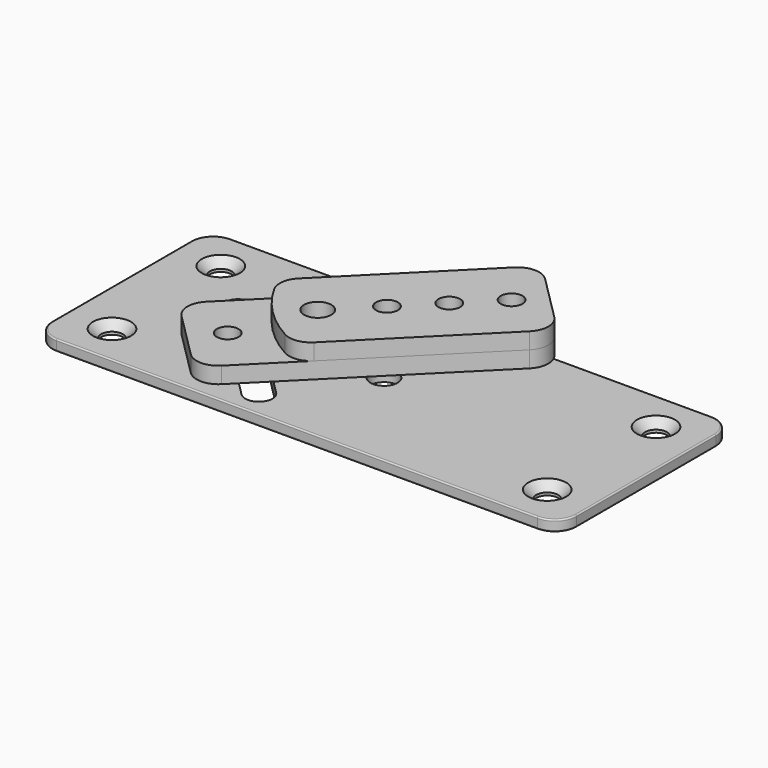
from build123d import *

# Parameters (mm, degrees)
F0_W      = 96.4
F0_H      = 2
F1_DEPTH  = 20
F2_R      = 4
F3_R      = 0.25
F4_R      = 2
F4_R_2    = 2.5
F5_DEPTH  = 2.0010001
F6_SIZE   = 1.5
F8_DEPTH  = 2.0010001
F9_R      = 2
F10_DEPTH = 3
F11_R     = 2.5
F11_R_2   = 2
F12_DEPTH = 3


# Not quite as in the source:
# - a feature names something its author has since deleted; it is built from what else it names


with BuildPart() as f1:
    # F0 (on Front) → F1 (new body, symmetric)
    with BuildSketch(Plane.XZ):
        with Locations((0, 1)):
            Rectangle(F0_W, F0_H)
    extrude(amount=F1_DEPTH, both=True)

    # F2
    f2_edges = [f1.edges().sort_by_distance(p)[0] for p in [
        (-48.2, -20, 1),
        (48.2, -20, 1),
        (48.2, 20, 1),
        (-48.2, 20, 1),
    ]]
    fillet(f2_edges, radius=F2_R)

    # F3
    f3_edges = [f1.edges().sort_by_distance(p)[0] for p in [
        (0, 20, 2),
        (47.028427, 18.828427, 2),
        (-47.028427, 18.828427, 2),
        (48.2, 0, 2),
        (-48.2, 0, 2),
        (47.028427, -18.828427, 2),
        (-47.028427, -18.828427, 2),
        (0, -20, 2),
        (-48.2, 0, 0),
        (-47.028427, 18.828427, 0),
        (-47.028427, -18.828427, 0),
        (0, 20, 0),
        (0, -20, 0),
        (47.028427, 18.828427, 0),
        (47.028427, -18.828427, 0),
        (48.2, 0, 0),
    ]]
    fillet(f3_edges, radius=F3_R)

    # F4 (on Top) → F5 (cut, through all)
    with BuildSketch(Plane.XY):
        with Locations((-40, 12.5)):
            Circle(F4_R)
        with Locations((-40, -12.5)):
            Circle(F4_R)
        with Locations((40, 12.5)):
            Circle(F4_R)
        with Locations((40, -12.5)):
            Circle(F4_R)
        Circle(F4_R_2)
    extrude(amount=F5_DEPTH, mode=Mode.SUBTRACT)

    # F6
    f6_edges = [f1.edges().sort_by_distance(p)[0] for p in [
        (-42, 12.5, 2),
        (-42, -12.5, 2),
        (38, -12.5, 2),
        (38, 12.5, 2),
    ]]
    chamfer(f6_edges, length=F6_SIZE)

    # F7 (on Top) → F8 (cut, through all)
    with BuildSketch(Plane.XY):
        with BuildLine():
            ThreePointArc((0, 13), (1.4142135624, 13.5857864376), (2, 15))
            ThreePointArc((2, 15), (-1.4142135624, 16.4142135624), (0, 13))
        make_face()
        with BuildLine():
            Line((-9.1768776335, -13.3023969122), (-28.3023969122, 5.8231223665))
            ThreePointArc((-28.3023969122, 5.8231223665), (-31.8379308181, 5.8231223665), (-31.8379308181, 2.2875884606))
            Line((-31.8379308181, 2.2875884606), (-12.7124115394, -16.8379308181))
            ThreePointArc((-12.7124115394, -16.8379308181), (-9.1768776335, -16.8379308181), (-9.1768776335, -13.3023969122))
        make_face()
    extrude(amount=F8_DEPTH, mode=Mode.SUBTRACT)


with BuildPart() as f10:
    # F9 (on face) → F10 (new body)
    with BuildSketch(Plane.XY.offset(2)):
        with BuildLine():
            Line((0.3535533906, 29.4956890143), (-31.1126983722, -1.9705627485))
            ThreePointArc((-31.1126983722, -1.9705627485), (-32.2842712475, -4.7989898732), (-31.1126983722, -7.627416998))
            Line((-31.1126983722, -7.627416998), (-22.627416998, -16.1126983722))
            ThreePointArc((-22.627416998, -16.1126983722), (-19.7989898732, -17.2842712475), (-16.9705627485, -16.1126983722))
            Line((-16.9705627485, -16.1126983722), (14.4956890143, 15.3535533906))
            ThreePointArc((14.4956890143, 15.3535533906), (15.6672618896, 18.1819805153), (14.4956890143, 21.0104076401))
            Line((14.4956890143, 21.0104076401), (6.0104076401, 29.4956890143))
            ThreePointArc((6.0104076401, 29.4956890143), (3.1819805153, 30.6672618896), (0.3535533906, 29.4956890143))
        make_face()
        with Locations((-22.627416998, -7.627416998)):
            Circle(F9_R, mode=Mode.SUBTRACT)
        with Locations((0, 15)):
            Circle(F9_R, mode=Mode.SUBTRACT)
    extrude(amount=F10_DEPTH)


with BuildPart() as f12:
    # F11 (on face) → F12 (new body)
    with BuildSketch(Plane.XY.offset(5)):
        with BuildLine():
            Line((0.3535533906, 29.4956890143), (-21.6698691325, 7.4722664912))
            ThreePointArc((-21.6698691325, 7.4722664912), (-22.8015135515, 5.2076064891), (-22.3468265674, 2.7171118067))
            ThreePointArc((-22.3468265674, 2.7171118067), (-18.0312229203, -3.0312229203), (-12.2828881933, -7.3468265674))
            ThreePointArc((-12.2828881933, -7.3468265674), (-9.7923935109, -7.8015135515), (-7.5277335088, -6.6698691325))
            Line((-7.5277335088, -6.6698691325), (14.4956890143, 15.3535533906))
            ThreePointArc((14.4956890143, 15.3535533906), (15.6672618896, 18.1819805153), (14.4956890143, 21.0104076401))
            Line((14.4956890143, 21.0104076401), (6.0104076401, 29.4956890143))
            ThreePointArc((6.0104076401, 29.4956890143), (3.1819805153, 30.6672618896), (0.3535533906, 29.4956890143))
        make_face()
        with Locations((-13.4350288425, 1.5649711575)):
            Circle(F11_R, mode=Mode.SUBTRACT)
        with Locations((-6.3639610307, 8.6360389693)):
            Circle(F11_R_2, mode=Mode.SUBTRACT)
        with Locations((0, 15)):
            Circle(F11_R_2, mode=Mode.SUBTRACT)
        with Locations((6.3639610307, 21.3639610307)):
            Circle(F11_R_2, mode=Mode.SUBTRACT)
    extrude(amount=F12_DEPTH)


solid = Compound([f1.part, f10.part, f12.part])
